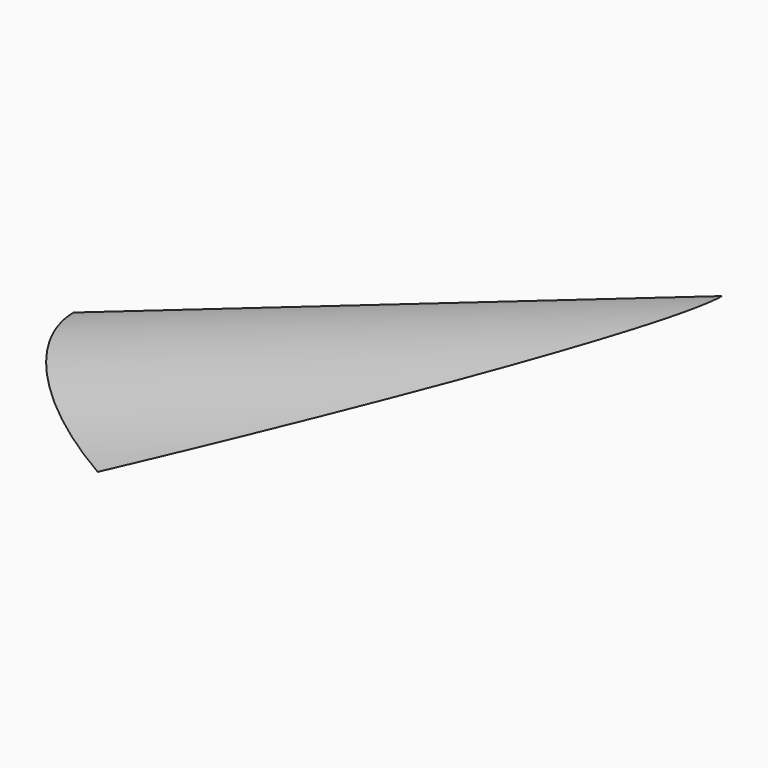
from build123d import *

# Parameters (mm, degrees)
F1_DEPTH    = 12.7
F2_T1_DEPTH = 266.661182443


# Not quite as in the source:
# - a fillet or chamfer that OpenCascade refuses, or shapes differently, is made with other operations: its cross-section is extruded or revolved along the edge and cut away or added


with BuildPart() as f1:
    # F0 (on Front) → F1 (new body, symmetric)
    with BuildSketch(Plane.XZ):
        Polygon((15.2311827987, 28.618497774), (-116.6892051697, -17.2318797559), (-92.2892913222, -27.9571134597), align=None)
    extrude(amount=F1_DEPTH, both=True)

    # F2: fillet of radius 25.4 on 1 edges, made by hand

    # F2_s2 → F2_t1 (cut)
    with BuildSketch(Plane(origin=(82.4446889798, 0, 28.6545557762), x_dir=(0, 1, 0), z_dir=(-0.9445744742, 0, -0.3282972171))):
        with BuildLine():
            ThreePointArc((12.7, -22.0319475609), (-5.2605122421, -14.592459803), (-12.7, 3.3680524391))
            Line((-12.7, 3.3680524391), (-12.7, -22.0319475609))
            Line((-12.7, -22.0319475609), (12.7, -22.0319475609))
        make_face()
    extrude(amount=F2_T1_DEPTH, mode=Mode.SUBTRACT)


solid = f1.part
